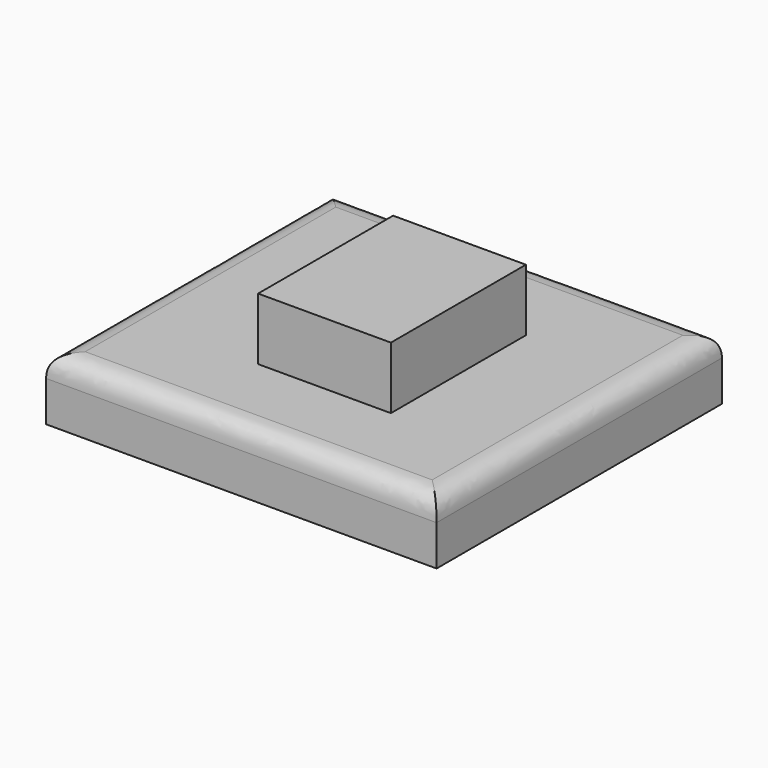
from build123d import *

# Parameters (mm, degrees)
F1_W        = 125.7533915341
F1_H        = 114.8591116071
F2_DEPTH    = 20
F3_T        = -5
F5_W        = 42.7649468184
F5_H        = 54.3430875987
F6_DEPTH    = 40
F7_T1_DEPTH = 149.8591116071
F7_T3_DEPTH = 160.7533915341


# Not quite as in the source:
# - a fillet or chamfer that OpenCascade refuses, or shapes differently, is made with other operations: its cross-section is extruded or revolved along the edge and cut away or added


with BuildPart() as f2:
    # F1 (on face) → F2 (new body)
    with BuildSketch(Plane.XY):
        with Locations((-2.1778326482, 3.7721171975)):
            Rectangle(F1_W, F1_H)
    extrude(amount=F2_DEPTH)

    # F3
    f3_openings = [f2.faces().sort_by_distance(p)[0] for p in [
        (-2.177833, 3.772117, 0),
    ]]
    offset(amount=F3_T, openings=f3_openings)

    # F5 (on Top) → F6 (join)
    with BuildSketch(Plane.XY):
        with Locations((1.4939792454, 2.4008983746)):
            Rectangle(F5_W, F5_H)
    extrude(amount=F6_DEPTH)

    # F7: fillet of radius 7 on 4 edges, made by hand

    # F7_s2 → F7_t1 (cut)
    with BuildSketch(Plane.XZ.offset(-78.7016730011)):
        with BuildLine():
            add(Edge.make_bspline(
                [(-58.0545284152, 20), (-65.0545284152, 20), (-65.0545284152, 13)],
                knots=[0, 0, 0, 1, 1, 1], degree=2, weights=[1, 1, 1]))
            Line((-65.0545284152, 13), (-65.0545284152, 20))
            Line((-65.0545284152, 20), (-58.0545284152, 20))
        make_face()
        with BuildLine():
            add(Edge.make_bspline(
                [(60.6988631189, 13), (60.6988631189, 20), (53.6988631189, 20)],
                knots=[0, 0, 0, 1, 1, 1], degree=2, weights=[1, 1, 1]))
            Line((53.6988631189, 20), (60.6988631189, 20))
            Line((60.6988631189, 20), (60.6988631189, 13))
        make_face()
    extrude(amount=F7_T1_DEPTH, mode=Mode.SUBTRACT)

    # F7_s4 → F7_t3 (cut)
    with BuildSketch(Plane.YZ.offset(-82.5545284152)):
        with BuildLine():
            add(Edge.make_bspline(
                [(-53.657438606, 13), (-53.657438606, 20), (-46.657438606, 20)],
                knots=[0, 0, 0, 1, 1, 1], degree=2, weights=[1, 1, 1]))
            Line((-46.657438606, 20), (-53.657438606, 20))
            Line((-53.657438606, 20), (-53.657438606, 13))
        make_face()
        with BuildLine():
            add(Edge.make_bspline(
                [(61.2016730011, 13), (61.2016730011, 20), (54.2016730011, 20)],
                knots=[0, 0, 0, 1, 1, 1], degree=2, weights=[1, 1, 1]))
            Line((54.2016730011, 20), (61.2016730011, 20))
            Line((61.2016730011, 20), (61.2016730011, 13))
        make_face()
    extrude(amount=F7_T3_DEPTH, mode=Mode.SUBTRACT)


solid = f2.part
